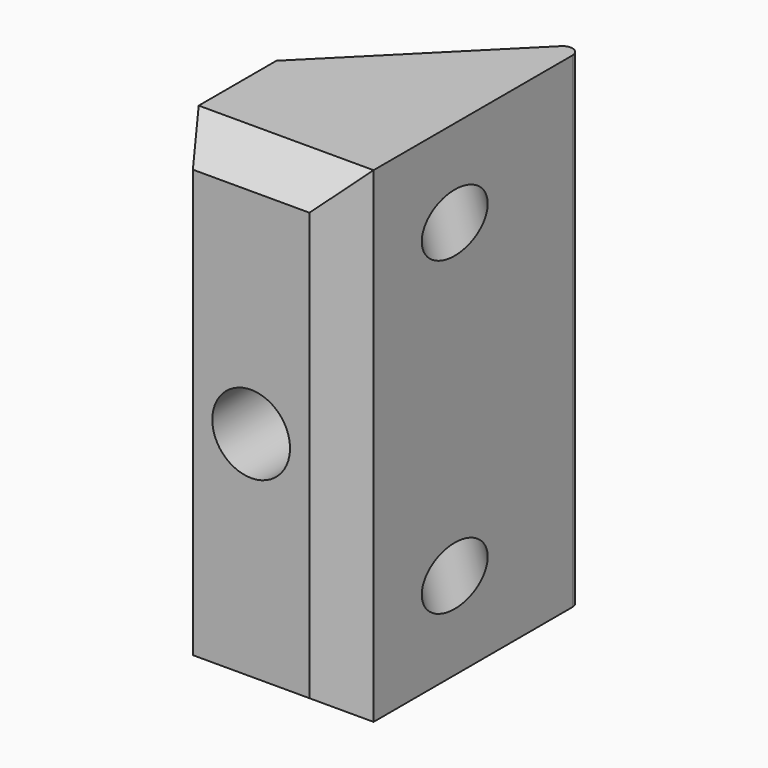
from build123d import *

# Parameters (mm, degrees)
F1_DEPTH = 25
F2_SIZE2 = 2.25
F2_SIZE  = 1.5
F4_D     = 4
F6_D     = 3
F9_D     = 7
F9_DEPTH = 7.5438932188


# Not quite as in the source:
# - a feature names something its author has since deleted; it is built from what else it names


with BuildPart() as f1:
    # F0 (on Top) → F1 (new body)
    with BuildSketch(Plane.XY):
        with BuildLine():
            Line((2.7078659423, 3.7500000373), (2.7078659423, 8.7500000373))
            Line((2.7078659423, 8.7500000373), (2.7078659423, 16.5428932561))
            ThreePointArc((2.7078659423, 16.5428932561), (2.3992076585, 17.0048330223), (1.8543125517, 16.8964466467))
            Line((1.8543125517, 16.8964466467), (-6.2921340577, 8.7500000373))
            Line((-6.2921340577, 8.7500000373), (-6.2921340577, 3.7500000373))
            Line((-6.2921340577, 3.7500000373), (-4.7921340577, 1.5000000373))
            Line((-4.7921340577, 1.5000000373), (1.2078659423, 1.5000000373))
            Line((1.2078659423, 1.5000000373), (2.7078659423, 3.7500000373))
        make_face()
    extrude(amount=F1_DEPTH)

    # F2
    f2_edges = [f1.edges().sort_by_distance(p)[0] for p in [
        (-1.792134, 1.5, 25),
        (-1.792134, 1.5, 0),
    ]]
    chamfer(f2_edges, length=F2_SIZE, length2=F2_SIZE2)

    # F4 (through all)
    with Locations(Plane.XZ.offset(-1.5000000373)):
        with Locations((-1.7921340577, 12.5)):
            Hole(F4_D / 2)

    # F6 (through all)
    with Locations(Plane(origin=(-7.5210670475, 7.5210670475, 0), x_dir=(-0.7071067812, -0.7071067812, 0), z_dir=(-0.7071067812, 0.7071067812, 0))):
        with Locations((-8.2587889815, 4.5), (-8.2587889815, 20.5)):
            Hole(F6_D / 2)

    # F9 (through all, one way)
    with BuildSketch(Plane.XZ.offset(-9.5000000373)):
        with Locations((-1.7921340577, 12.5)):
            Circle(F9_D / 2)
    extrude(amount=-F9_DEPTH, mode=Mode.SUBTRACT)


solid = f1.part
